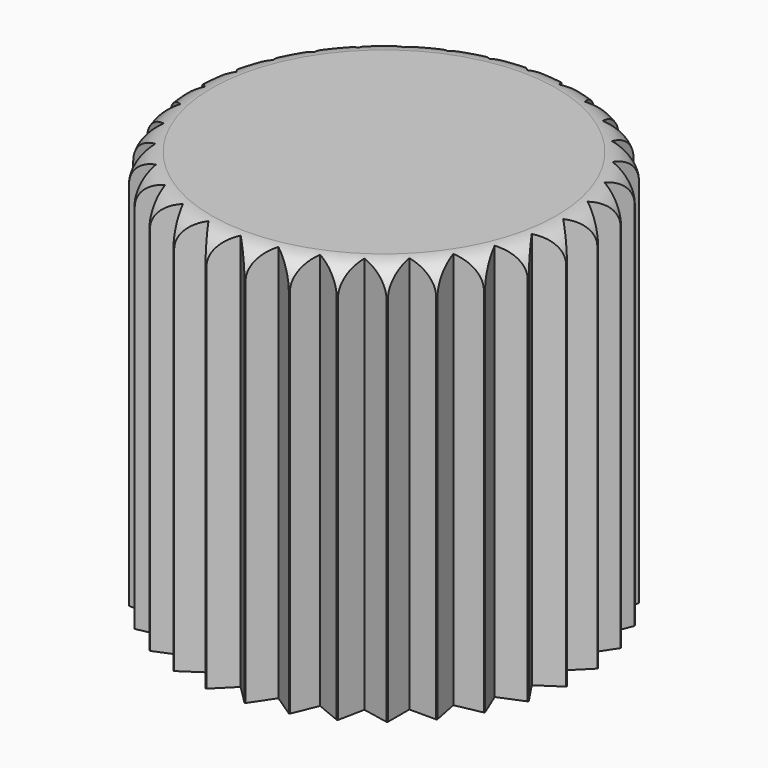
from build123d import *

# Parameters (mm, degrees)
F0_R            = 7.5
F1_DEPTH        = 15
F2_R            = 5.25
F3_DEPTH        = 5.6
F5_R            = 1
F6_DEPTH        = 5.6
F9_DEPTH        = 15.001
F9_COPIES_COUNT = 32
F10_DEPTH       = 2.2


# Not quite as in the source:
# - a pattern or mirror of a feature is missing from the dataset's text; its kind, count and spacing are read off the source's solid


with BuildPart() as f1:
    # F0 (on Top) → F1 (new body)
    with BuildSketch(Plane.XY):
        Circle(F0_R)
    extrude(amount=F1_DEPTH)

    # F2 (on Top) → F3 (cut)
    with BuildSketch(Plane.XY):
        Circle(F2_R)
    extrude(amount=F3_DEPTH, mode=Mode.SUBTRACT)

    # F5
    f5_edges = [f1.edges().sort_by_distance(p)[0] for p in [
        (-7.5, 0, 15),
    ]]
    fillet(f5_edges, radius=F5_R)

    # F4 (on Top) → F6 (join, through all)
    with BuildSketch(Plane.XY):
        Polygon((-2.8867513459, 0), (-1.443375673, -2.5), (1.443375673, -2.5), (2.8867513459, 0), (1.443375673, 2.5), (-1.443375673, 2.5), align=None)
    extrude(amount=F6_DEPTH)

    # F7 (on face) → F9 (cut, through all)
    with BuildSketch(Plane.XY.offset(15)):
        with BuildLine():
            Line((0, -6.75), (-0.715767043, -7.465767043))
            ThreePointArc((-0.715767043, -7.465767043), (0, -7.5), (0.715767043, -7.465767043))
            Line((0.715767043, -7.465767043), (0, -6.75))
        make_face()
    f9 = extrude(amount=-F9_DEPTH, mode=Mode.SUBTRACT)

    # F9_copies: F9 ×32 about axis
    f9_copies_axis = Axis((0, 0, 0), (0, 0, 1))
    for i in range(1, F9_COPIES_COUNT):
        add(f9.rotate(f9_copies_axis, i * 360 / F9_COPIES_COUNT), mode=Mode.SUBTRACT)

    # F10 (cut): a face of the model
    f10_faces = [f1.faces().sort_by_distance(p)[0] for p in [
        (0, 0, 0),
    ]]
    extrude(f10_faces, amount=-F10_DEPTH, mode=Mode.SUBTRACT)


solid = f1.part
